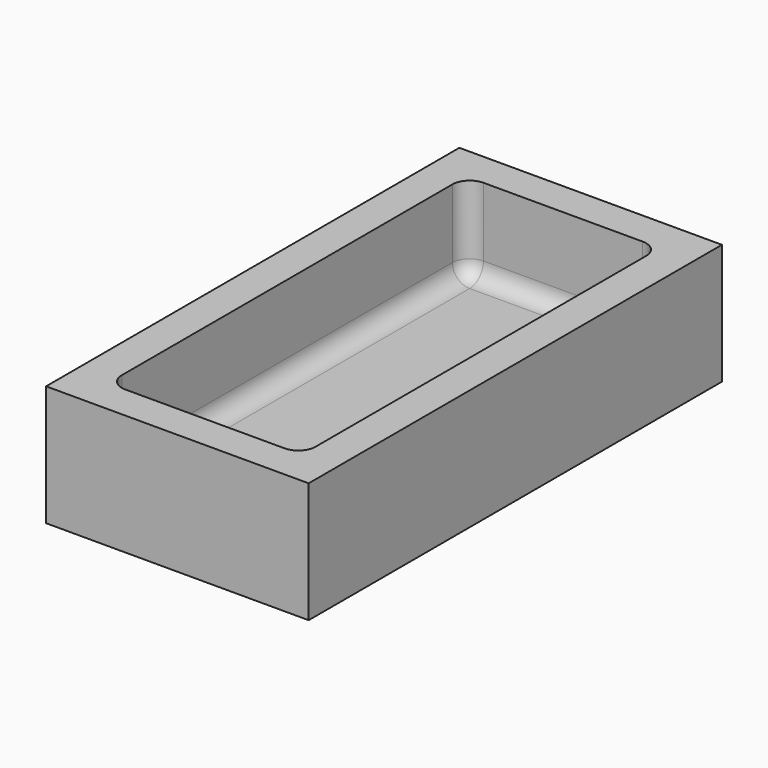
from build123d import *

# Parameters (mm, degrees)
F0_W     = 774.7
F0_H     = 1524
F1_DEPTH = 355.6
F2_T     = -101.6
F3_R     = 50.8


with BuildPart() as f1:
    # F0 (on Top) → F1 (new body)
    with BuildSketch(Plane.XY):
        with Locations((-694.7045188031, -13.3193368092)):
            Rectangle(F0_W, F0_H)
    extrude(amount=F1_DEPTH)

    # F2
    f2_openings = [f1.faces().sort_by_distance(p)[0] for p in [
        (-694.704519, -13.319337, 355.6),
    ]]
    offset(amount=F2_T, openings=f2_openings)

    # F3
    f3_edges = [f1.edges().sort_by_distance(p)[0] for p in [
        (-980.454519, -13.319337, 101.6),
        (-694.704519, -673.719337, 101.6),
        (-408.954519, -13.319337, 101.6),
        (-694.704519, 647.080663, 101.6),
        (-408.954519, -673.719337, 228.6),
        (-408.954519, 647.080663, 228.6),
        (-980.454519, 647.080663, 228.6),
        (-980.454519, -673.719337, 228.6),
    ]]
    fillet(f3_edges, radius=F3_R)


solid = f1.part
